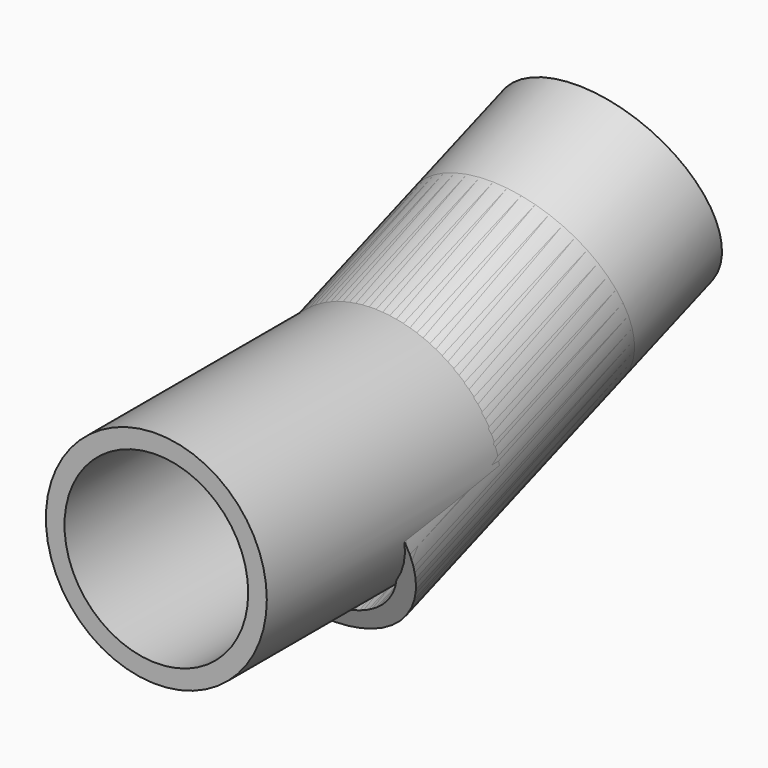
from build123d import *
from build123d import SkipClean  # not in build123d's __all__

# Parameters (mm, degrees)
F0_R          = 9.5
F0_R_2        = 7.9
F1_DEPTH      = 25
F4_R          = 9.5
F4_R_2        = 7.9
F5_DEPTH      = 25
F5_DEPTH_BACK = 10
F6_DEPTH      = 25


with BuildPart() as f1:
    # F0 (on Front) → F1 (new body)
    with BuildSketch(Plane.XZ):
        Circle(F0_R)
        Circle(F0_R_2, mode=Mode.SUBTRACT)
    extrude(amount=F1_DEPTH)



with BuildPart() as f5:
    # F4 (on face) → F5 (new body, two sides)
    with BuildSketch(Plane(origin=(0, 0, 0), x_dir=(-1, 0, 0), z_dir=(0, 0.9396926208, 0.3420201433))) as f5_sk:
        Circle(F4_R)
        Circle(F4_R_2, mode=Mode.SUBTRACT)
    extrude(amount=F5_DEPTH)
    extrude(f5_sk.sketch, amount=-F5_DEPTH_BACK)


with BuildPart() as f1_1:
    add(f1.part, clean=False)
    # F6 (add): a face of the model
    f6_faces = [f5.part.faces().sort_by_distance(p)[0] for p in [
        (9.2312994231, -9.3969262079, -3.4202014333),
    ]]
    with SkipClean():  # cleaning this boolean's faces spoils the solid; the shape is the same uncleaned
        extrude(f6_faces, amount=-F6_DEPTH)


solid = Compound([f5.part, f1_1.part])
